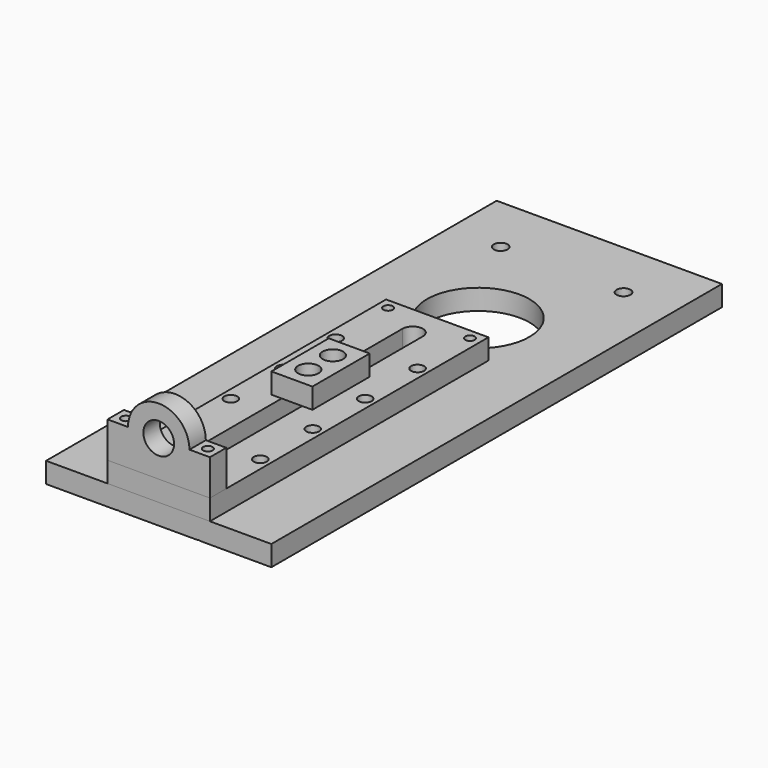
from build123d import *

# Parameters (mm, degrees)
F2_W             = 69.85
F2_H             = 174.625
F2_R             = 2.15265
F2_R_2           = 15.875
F3_DEPTH         = 6.35
F4_W             = 31.75
F4_H             = 107.95
F5_DEPTH         = 6.35
F6_D             = 4.0386
F7_R             = 4.7625
F8_DEPTH         = 6.35
F9_D             = 2.9464
F9_CSINK_D       = 6.477
F9_CSINK_ANGLE   = 82
F9_2_D           = 2.9464
F9_2_CSINK_D     = 6.477
F9_2_CSINK_ANGLE = 82
F9_3_D           = 2.9464
F9_3_CSINK_D     = 6.477
F9_3_CSINK_ANGLE = 82
F10_W            = 12.7
F10_H            = 22.225
F10_R            = 3.175
F11_DEPTH        = 6.35


# Not quite as in the source:
# - a variable given as a bare number and used for a length is read in inches; the dataset says mm whatever the document's units were


with BuildPart() as f3:
    # F2 (on Top) → F3 (new body)
    with BuildSketch(Plane.XY):
        Rectangle(F2_W, F2_H)
        with BuildLine():
            ThreePointArc((-5.55625, 11.1125), (0, 16.66875), (5.55625, 11.1125))
            Line((5.55625, 11.1125), (5.55625, -77.7875))
            ThreePointArc((5.55625, -77.7875), (0, -83.34375), (-5.55625, -77.7875))
            Line((-5.55625, -77.7875), (-5.55625, 11.1125))
        make_face(mode=Mode.SUBTRACT)
        with Locations((-19.05, 69.0245)):
            Circle(F2_R, mode=Mode.SUBTRACT)
        with Locations((0, 36.5125)):
            Circle(F2_R_2, mode=Mode.SUBTRACT)
        with Locations((19.05, 69.0245)):
            Circle(F2_R, mode=Mode.SUBTRACT)
    extrude(amount=F3_DEPTH)

    # F9 (through all)
    with Locations(Plane(origin=(0, 0, 0), x_dir=(1, 0, 0), z_dir=(0, 0, -1))):
        with Locations((12.7, 84.1375), (-12.7, 84.1375), (-12.7, -17.4625), (12.7, -17.4625)):
            CounterSinkHole(F9_D / 2, F9_CSINK_D / 2, counter_sink_angle=F9_CSINK_ANGLE)


with BuildPart() as f5:
    # F4 (on face) → F5 (new body)
    with BuildSketch(Plane.XY.offset(6.35)):
        with Locations((0, -33.3375)):
            Rectangle(F4_W, F4_H)
        with BuildLine():
            ThreePointArc((-3.175, 11.1125), (0, 14.2875), (3.175, 11.1125))
            Line((3.175, 11.1125), (3.175, -77.7875))
            ThreePointArc((3.175, -77.7875), (0, -80.9625), (-3.175, -77.7875))
            Line((-3.175, -77.7875), (-3.175, 11.1125))
        make_face(mode=Mode.SUBTRACT)
    extrude(amount=F5_DEPTH)

    # F6 (through all)
    with Locations(Plane(origin=(0, 0, 6.35), x_dir=(1, 0, 0), z_dir=(0, 0, -1))):
        with Locations((-12.7, 63.8175), (-12.7, 43.4975), (-12.7, 23.1775), (-12.7, 2.8575), (12.7, 2.8575), (12.7, 23.1775), (12.7, 43.4975), (12.7, 63.8175)):
            Hole(F6_D / 2)

    # F9#2 (through all)
    with Locations(Plane(origin=(0, 0, 0), x_dir=(1, 0, 0), z_dir=(0, 0, -1))):
        with Locations((12.7, 84.1375), (-12.7, 84.1375), (-12.7, -17.4625), (12.7, -17.4625)):
            CounterSinkHole(F9_2_D / 2, F9_2_CSINK_D / 2, counter_sink_angle=F9_2_CSINK_ANGLE)


with BuildPart() as f8:
    # F7 (on face) → F8 (new body)
    with BuildSketch(Plane.XZ.offset(87.3125)):
        with BuildLine():
            Line((-15.875, 23.84425), (-15.875, 12.7))
            Line((-15.875, 12.7), (15.875, 12.7))
            Line((15.875, 12.7), (15.875, 23.84425))
            Line((15.875, 23.84425), (9.525, 23.84425))
            ThreePointArc((9.525, 23.84425), (0, 33.36925), (-9.525, 23.84425))
            Line((-9.525, 23.84425), (-15.875, 23.84425))
        make_face()
        with Locations((0, 23.84425)):
            Circle(F7_R, mode=Mode.SUBTRACT)
    extrude(amount=-F8_DEPTH)

    # F9#3 (through all)
    with Locations(Plane(origin=(0, 0, 0), x_dir=(1, 0, 0), z_dir=(0, 0, -1))):
        with Locations((12.7, 84.1375), (-12.7, 84.1375), (-12.7, -17.4625), (12.7, -17.4625)):
            CounterSinkHole(F9_3_D / 2, F9_3_CSINK_D / 2, counter_sink_angle=F9_3_CSINK_ANGLE)


with BuildPart() as f11:
    # F10 (on face) → F11 (new body)
    with BuildSketch(Plane.XY.offset(12.7)):
        with Locations((0, -24.5792828321)):
            Rectangle(F10_W, F10_H)
        with Locations((0, -29.3417828321)):
            Circle(F10_R, mode=Mode.SUBTRACT)
        with Locations((0, -19.8167828321)):
            Circle(F10_R, mode=Mode.SUBTRACT)
    extrude(amount=F11_DEPTH)


solid = Compound([f3.part, f5.part, f8.part, f11.part])
